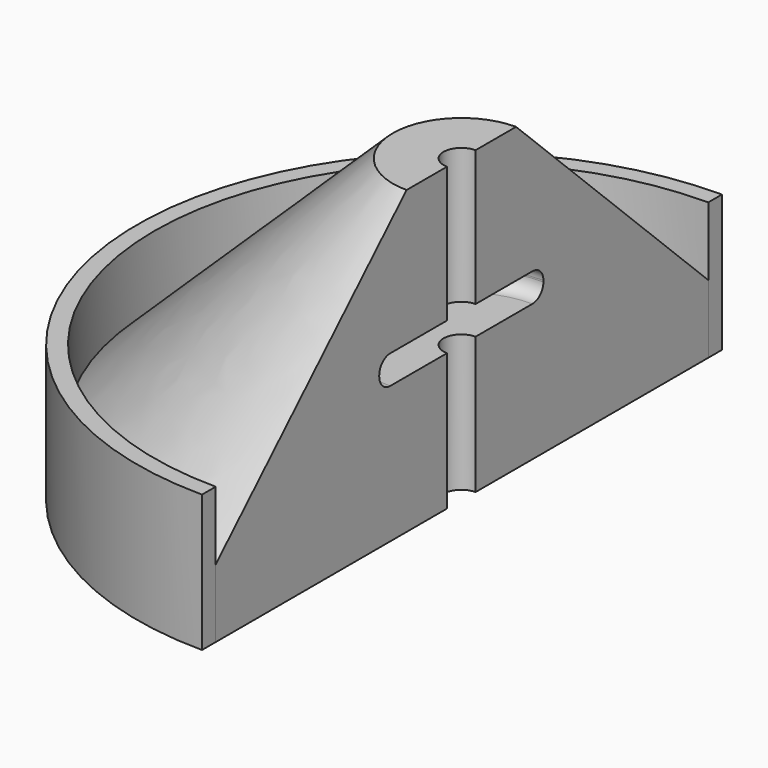
from build123d import *

# Parameters (mm, degrees)
F1_DEPTH  = 25.4
F2_DEPTH  = 50.8
F9_R      = 6.604
F10_DEPTH = 111.76
F11_R     = 38.1
F12_DEPTH = 10.668
F13_R     = 5.08


with BuildPart() as f1:
    # F0 (on Top) → F1 (new body)
    with BuildSketch(Plane.XY):
        with BuildLine():
            Line((0, -114.0008171796), (0, 114.599125499))
            ThreePointArc((0, 114.599125499), (-114.2190565937, 0.2991541597), (0, -114.0008171796))
        make_face()
    extrude(amount=F1_DEPTH)

    # F0 (on Top) → F2 (join)
    with BuildSketch(Plane.XY):
        with BuildLine():
            ThreePointArc((0, -114.0008171796), (-114.2190565937, 0.2991541597), (0, 114.599125499))
            Line((0, 114.599125499), (-0.0044968559, 120.9491239067))
            ThreePointArc((-0.0044968559, 120.9491239067), (-120.5690565937, 0.2991541597), (-0.0044968559, -120.3508155874))
            Line((-0.0044968559, -120.3508155874), (0, -114.0008171796))
        make_face()
    extrude(amount=F2_DEPTH)

    # F1_face (on face) → F5 section 0
    with BuildSketch(Plane(origin=(-48.4732263634, 0.2991541597, 25.4), x_dir=(1, 0, 0), z_dir=(0, 0, 1))):
        with BuildLine():
            Line((48.4732263634, -114.2999713393), (48.4732263634, 114.2999713393))
            ThreePointArc((48.4732263634, 114.2999713393), (-65.7458302303, 0), (48.4732263634, -114.2999713393))
        make_face()
    # F4 (on offset) → F5 section 1
    with BuildSketch(Plane.XY.offset(111.76)):
        with BuildLine():
            Line((0, 0), (0, 25.4))
            ThreePointArc((0, 25.4), (-25.4, 0), (0, -25.4))
            Line((0, -25.4), (0, 0))
        make_face()
    loft()

    # F9 (on Top) → F10 (cut)
    with BuildSketch(Plane.XY):
        Circle(F9_R)
    extrude(amount=F10_DEPTH, mode=Mode.SUBTRACT)

    # F11 (on offset) → F12 (cut)
    with BuildSketch(Plane.XY.offset(50.8)):
        Circle(F11_R)
    extrude(amount=F12_DEPTH, mode=Mode.SUBTRACT)

    # F13
    f13_edges = [f1.edges().sort_by_distance(p)[0] for p in [
        (-38.1, 0, 61.468),
        (-38.1, 0, 50.8),
    ]]
    fillet(f13_edges, radius=F13_R)


solid = f1.part
